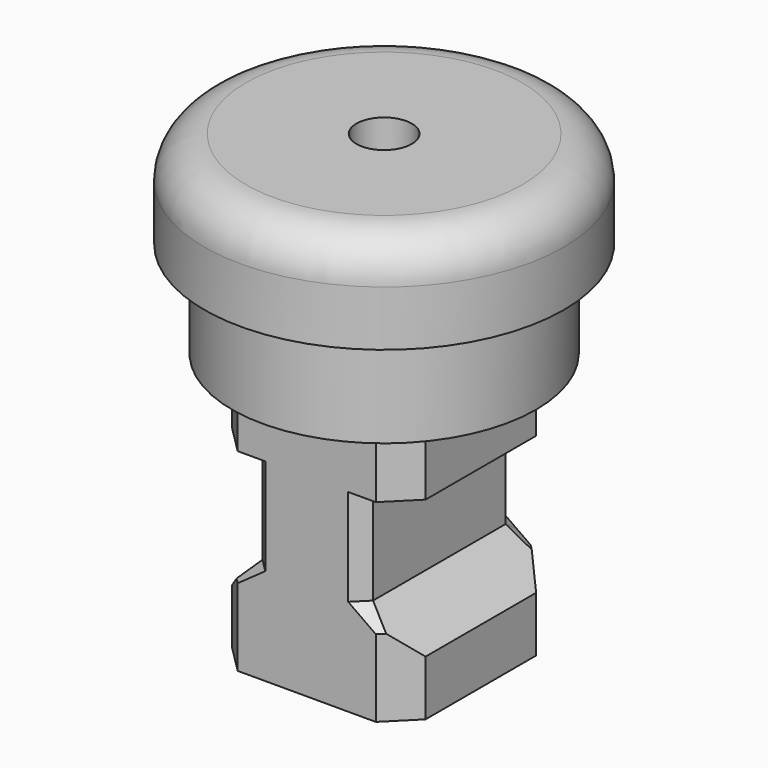
from build123d import *

# Parameters (mm, degrees)
F3_DEPTH     = 3.5
F4_SIZE      = 1
F5_SIZE      = 0.5
F6_T4_DEPTH  = 8.4221557451
F6_T11_DEPTH = 13.7150489639
F6_T21_DEPTH = 8.4221557451
F6_T28_DEPTH = 8.4221557451
F6_T35_DEPTH = 13.7150489639
F6_T45_DEPTH = 8.4221557451
F7_R         = 1.5
F8_R         = 1
F9_DEPTH     = 25


# Not quite as in the source:
# - a fillet or chamfer that OpenCascade refuses, or shapes differently, is made with other operations: its cross-section is extruded or revolved along the edge and cut away or added


with BuildPart() as f1:
    # F0 (on Front) → F1 (revolve)
    with BuildSketch(Plane.XZ):
        Polygon((0, 7), (0, 0), (5.5, 0), (5.5, 3.5), (6.5, 3.5), (6.5, 7), align=None)
    revolve(axis=Axis((0, 0, 5.0261294236), (0, 0, 1)))

    # F2 (on Front) → F3 (join, symmetric)
    with BuildSketch(Plane.XZ):
        Polygon((3.5, 0), (-3.5, 0), (-3.5, -2.5), (-2, -2.5), (-2, -7.5), (-3.5, -7.5), (-3.5, -9.5), (3.5, -9.5), (3.5, -7.5), (2, -7.5), (2, -2.5), (3.5, -2.5), align=None)
    extrude(amount=F3_DEPTH, both=True)

    # F4
    f4_edges = [f1.edges().sort_by_distance(p)[0] for p in [
        (3.5, -3.5, -1.25),
        (3.5, 3.5, -1.25),
        (-3.5, 3.5, -1.25),
        (-3.5, -3.5, -1.25),
        (-3.5, -3.5, -8.5),
        (3.5, -3.5, -8.5),
        (-3.5, 3.5, -8.5),
        (3.5, 3.5, -8.5),
    ]]
    chamfer(f4_edges, length=F4_SIZE)

    # F5
    f5_edges = [f1.edges().sort_by_distance(p)[0] for p in [
        (2, -3.5, -5),
        (-2, -3.5, -5),
        (-2, 3.5, -5),
        (2, 3.5, -5),
    ]]
    chamfer(f5_edges, length=F5_SIZE)

    # F6: chamfer of 1.5 on 6 edges, made by hand


with BuildPart() as f6_tool2:
    # F6_s3 → F6_t4 (new body)
    with BuildSketch(Plane(origin=(3.7276817198, -3.7276817198, 0), x_dir=(0, 0, 1), z_dir=(-0.7071067812, 0.7071067812, 0))):
        Polygon((-7.5, -5.0355339059), (-6, -3.5355339059), (-7.5, -3.5355339059), align=None)
    extrude(amount=F6_T4_DEPTH)

    split(bisect_by=Plane.XZ.offset(3.5), keep=Keep.BOTTOM)

    split(bisect_by=Plane(origin=(-3, -3, 0), x_dir=(0, 0, 1), z_dir=(0.7071067812, 0.7071067812, 0)), keep=Keep.TOP)

    split(bisect_by=Plane(origin=(2, 0, -2), x_dir=(0, 1, 0), z_dir=(0.7071067812, 0, -0.7071067812)), keep=Keep.TOP)


with BuildPart() as f1_1:
    add(f1.part)

    # F6_t1: union F6_tool2
    add(f6_tool2.part)


with BuildPart() as f6_tool9:
    # F6_s10 → F6_t11 (new body)
    with BuildSketch(Plane.XZ.offset(-6.8575244819)):
        Polygon((-3.5, -7.5), (-2, -6), (-2, -7.5), align=None)
    extrude(amount=F6_T11_DEPTH)

    split(bisect_by=Plane.XZ.offset(3.5), keep=Keep.BOTTOM)

    split(bisect_by=Plane(origin=(-3, -3, 0), x_dir=(0, 0, 1), z_dir=(0.7071067812, 0.7071067812, 0)), keep=Keep.TOP)

    split(bisect_by=Plane.XZ.offset(-3.5), keep=Keep.TOP)

    split(bisect_by=Plane(origin=(-3, 3, 0), x_dir=(0, 0, 1), z_dir=(0.7071067812, -0.7071067812, 0)), keep=Keep.TOP)

    split(bisect_by=Plane(origin=(0.8713203436, -0.8713203436, -1.232233047), x_dir=(0.7071067812, 0.7071067812, 0), z_dir=(0.5, -0.5, -0.7071067812)), keep=Keep.TOP)

    split(bisect_by=Plane(origin=(0.8713203436, 0.8713203436, -1.232233047), x_dir=(-0.7071067812, 0.7071067812, 0), z_dir=(0.5, 0.5, -0.7071067812)), keep=Keep.TOP)


with BuildPart() as f1_2:
    add(f1_1.part)

    # F6_t8: union F6_tool9
    add(f6_tool9.part)


with BuildPart() as f6_tool19:
    # F6_s20 → F6_t21 (new body)
    with BuildSketch(Plane(origin=(3.7276817198, 3.7276817198, 0), x_dir=(0, 0, 1), z_dir=(-0.7071067812, -0.7071067812, 0))):
        Polygon((-7.5, 5.0355339059), (-6, 3.5355339059), (-7.5, 3.5355339059), align=None)
    extrude(amount=F6_T21_DEPTH)

    split(bisect_by=Plane.XZ.offset(-3.5), keep=Keep.TOP)

    split(bisect_by=Plane(origin=(-3, 3, 0), x_dir=(0, 0, 1), z_dir=(0.7071067812, -0.7071067812, 0)), keep=Keep.TOP)

    split(bisect_by=Plane(origin=(2, 0, -2), x_dir=(0, 1, 0), z_dir=(0.7071067812, 0, -0.7071067812)), keep=Keep.TOP)


with BuildPart() as f1_3:
    add(f1_2.part)

    # F6_t18: union F6_tool19
    add(f6_tool19.part)


with BuildPart() as f6_tool26:
    # F6_s27 → F6_t28 (new body)
    with BuildSketch(Plane(origin=(-3.7276817198, -3.7276817198, 0), x_dir=(0, 0, 1), z_dir=(0.7071067812, 0.7071067812, 0))):
        Polygon((-7.5, 5.0355339059), (-6, 3.5355339059), (-7.5, 3.5355339059), align=None)
    extrude(amount=F6_T28_DEPTH)

    split(bisect_by=Plane.XZ.offset(3.5), keep=Keep.BOTTOM)

    split(bisect_by=Plane(origin=(3, -3, 0), x_dir=(0, 0, 1), z_dir=(-0.7071067812, 0.7071067812, 0)), keep=Keep.TOP)

    split(bisect_by=Plane(origin=(-2, 0, -2), x_dir=(0, 1, 0), z_dir=(-0.7071067812, 0, -0.7071067812)), keep=Keep.TOP)


with BuildPart() as f1_4:
    add(f1_3.part)

    # F6_t25: union F6_tool26
    add(f6_tool26.part)


with BuildPart() as f6_tool33:
    # F6_s34 → F6_t35 (new body)
    with BuildSketch(Plane.XZ.offset(-6.8575244819)):
        Polygon((3.5, -7.5), (2, -6), (2, -7.5), align=None)
    extrude(amount=F6_T35_DEPTH)

    split(bisect_by=Plane.XZ.offset(3.5), keep=Keep.BOTTOM)

    split(bisect_by=Plane(origin=(3, -3, 0), x_dir=(0, 0, 1), z_dir=(-0.7071067812, 0.7071067812, 0)), keep=Keep.TOP)

    split(bisect_by=Plane.XZ.offset(-3.5), keep=Keep.TOP)

    split(bisect_by=Plane(origin=(3, 3, 0), x_dir=(0, 0, 1), z_dir=(-0.7071067812, -0.7071067812, 0)), keep=Keep.TOP)

    split(bisect_by=Plane(origin=(-0.8713203436, -0.8713203436, -1.232233047), x_dir=(0.7071067812, -0.7071067812, 0), z_dir=(-0.5, -0.5, -0.7071067812)), keep=Keep.TOP)

    split(bisect_by=Plane(origin=(-0.8713203436, 0.8713203436, -1.232233047), x_dir=(-0.7071067812, -0.7071067812, 0), z_dir=(-0.5, 0.5, -0.7071067812)), keep=Keep.TOP)


with BuildPart() as f1_5:
    add(f1_4.part)

    # F6_t32: union F6_tool33
    add(f6_tool33.part)


with BuildPart() as f6_tool43:
    # F6_s44 → F6_t45 (new body)
    with BuildSketch(Plane(origin=(-3.7276817198, 3.7276817198, 0), x_dir=(0, 0, 1), z_dir=(0.7071067812, -0.7071067812, 0))):
        Polygon((-7.5, -5.0355339059), (-6, -3.5355339059), (-7.5, -3.5355339059), align=None)
    extrude(amount=F6_T45_DEPTH)

    split(bisect_by=Plane.XZ.offset(-3.5), keep=Keep.TOP)

    split(bisect_by=Plane(origin=(3, 3, 0), x_dir=(0, 0, 1), z_dir=(-0.7071067812, -0.7071067812, 0)), keep=Keep.TOP)

    split(bisect_by=Plane(origin=(-2, 0, -2), x_dir=(0, 1, 0), z_dir=(-0.7071067812, 0, -0.7071067812)), keep=Keep.TOP)


with BuildPart() as f1_6:
    add(f1_5.part)

    # F6_t42: union F6_tool43
    add(f6_tool43.part)

    # F7
    f7_edges = [f1_6.edges().sort_by_distance(p)[0] for p in [
        (-6.5, 0, 7),
    ]]
    fillet(f7_edges, radius=F7_R)

    # F8 (on face) → F9 (cut)
    with BuildSketch(Plane(origin=(0, 0, -9.5), x_dir=(1, 0, 0), z_dir=(0, 0, -1))):
        Circle(F8_R)
    extrude(amount=-F9_DEPTH, mode=Mode.SUBTRACT)


solid = f1_6.part
